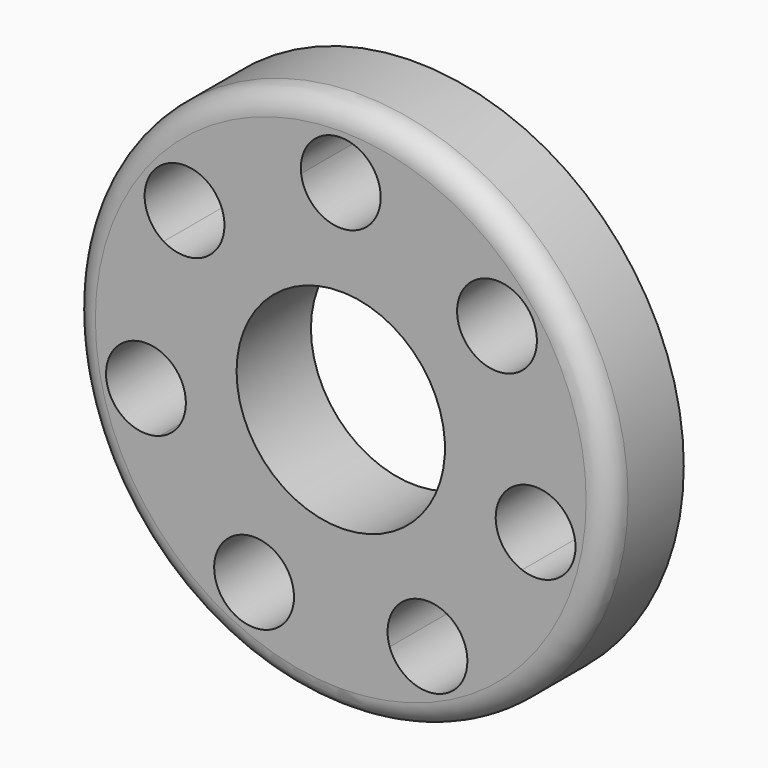
from build123d import *

# Parameters (mm, degrees)
F0_R     = 73.4225499851
F1_DEPTH = 25.4
F3_R     = 6.35
F5_DEPTH = 25.4
F6_R     = 28.4745991817
F7_DEPTH = 25.4


with BuildPart() as f1:
    # F0 (on Front) → F1 (new body)
    with BuildSketch(Plane.XZ):
        Circle(F0_R)
    extrude(amount=F1_DEPTH)

    # F3
    f3_edges = [f1.edges().sort_by_distance(p)[0] for p in [
        (-73.42255, -25.4, 0),
    ]]
    fillet(f3_edges, radius=F3_R)

    # F4 (on face) → F5 (cut)
    with BuildSketch(Plane.XZ.offset(25.4)):
        with BuildLine():
            ThreePointArc((10.828438703, 53.2833849069), (10.8892176697, 53.9458802451), (10.9095024699, 54.6108484268))
            ThreePointArc((10.9095024699, 54.6108484268), (-0.6649681817, 65.5000660965), (-10.828438703, 53.2833849069))
            ThreePointArc((-10.828438703, 53.2833849069), (0, 54.3725499851), (10.828438703, 53.2833849069))
        make_face()
        with BuildLine():
            ThreePointArc((10.828438703, 53.2833849069), (0, 54.3725499851), (-10.828438703, 53.2833849069))
            ThreePointArc((-10.828438703, 53.2833849069), (0, 43.7013459569), (10.828438703, 53.2833849069))
        make_face()
        with BuildLine():
            ThreePointArc((-48.4100489141, 24.7556328141), (-42.5101713604, 33.9007304168), (-34.9072067114, 41.6876613819))
            ThreePointArc((-34.9072067114, 41.6876613819), (-51.2258730734, 40.8512705983), (-48.4100489141, 24.7556328141))
        make_face()
        with BuildLine():
            ThreePointArc((-31.7869781145, 34.049307065), (-32.5971155871, 38.1748459137), (-34.9072067114, 41.6876613819))
            ThreePointArc((-34.9072067114, 41.6876613819), (-42.5101713604, 33.9007304168), (-48.4100489141, 24.7556328141))
            ThreePointArc((-48.4100489141, 24.7556328141), (-37.3727104759, 24.5269798299), (-31.7869781145, 34.049307065))
        make_face()
        with BuildLine():
            ThreePointArc((48.4100489141, 24.7556328141), (42.5101713604, 33.9007304168), (34.9072067114, 41.6876613819))
            ThreePointArc((34.9072067114, 41.6876613819), (34.1670880954, 27.2473435317), (48.4100489141, 24.7556328141))
        make_face()
        with BuildLine():
            ThreePointArc((53.6059830542, 34.049307065), (46.8220194331, 44.1486720622), (34.9072067114, 41.6876613819))
            ThreePointArc((34.9072067114, 41.6876613819), (42.5101713604, 33.9007304168), (48.4100489141, 24.7556328141))
            ThreePointArc((48.4100489141, 24.7556328141), (52.2188078195, 28.7255369565), (53.6059830542, 34.049307065))
        make_face()
        with BuildLine():
            ThreePointArc((-49.5379049078, -22.4136157107), (-53.009316637, -12.0990306043), (-54.3570134948, -1.299721437))
            ThreePointArc((-54.3570134948, -1.299721437), (-63.8776189051, -14.5796496747), (-49.5379049078, -22.4136157107))
        make_face()
        with BuildLine():
            ThreePointArc((-42.3321379694, -12.1520569961), (-45.9324312127, -4.0531246824), (-54.3570134948, -1.299721437))
            ThreePointArc((-54.3570134948, -1.299721437), (-53.009316637, -12.0990306043), (-49.5379049078, -22.4136157107))
            ThreePointArc((-49.5379049078, -22.4136157107), (-44.3135063658, -18.421480104), (-42.3321379694, -12.1520569961))
        make_face()
        with BuildLine():
            ThreePointArc((49.5379049078, -22.4136157107), (53.009316637, -12.0990306043), (54.3570134948, -1.299721437))
            ThreePointArc((54.3570134948, -1.299721437), (42.6056619733, -9.7244643175), (49.5379049078, -22.4136157107))
        make_face()
        with BuildLine():
            ThreePointArc((64.1511429091, -12.1520569961), (61.340572753, -4.8428477695), (54.3570134948, -1.299721437))
            ThreePointArc((54.3570134948, -1.299721437), (53.009316637, -12.0990306043), (49.5379049078, -22.4136157107))
            ThreePointArc((49.5379049078, -22.4136157107), (59.5110635472, -21.0801910696), (64.1511429091, -12.1520569961))
        make_face()
        with BuildLine():
            ThreePointArc((-13.3627081169, -52.7049544509), (-23.5913652929, -48.9879748051), (-32.8748804356, -43.3083875044))
            ThreePointArc((-32.8748804356, -43.3083875044), (-28.4282148354, -59.031796372), (-13.3627081169, -52.7049544509))
        make_face()
        with BuildLine():
            ThreePointArc((-12.7852566419, -49.2026742823), (-20.6233841848, -38.7344413752), (-32.8748804356, -43.3083875044))
            ThreePointArc((-32.8748804356, -43.3083875044), (-23.5913652929, -48.9879748051), (-13.3627081169, -52.7049544509))
            ThreePointArc((-13.3627081169, -52.7049544509), (-12.930587523, -50.9774571271), (-12.7852566419, -49.2026742823))
        make_face()
        with BuildLine():
            ThreePointArc((13.3627081169, -52.7049544509), (23.5913652929, -48.9879748051), (32.8748804356, -43.3083875044))
            ThreePointArc((32.8748804356, -43.3083875044), (18.9613033883, -39.3735521926), (13.3627081169, -52.7049544509))
        make_face()
        with BuildLine():
            ThreePointArc((34.6042615817, -49.2026742823), (34.1629920189, -46.1312993553), (32.8748804356, -43.3083875044))
            ThreePointArc((32.8748804356, -43.3083875044), (23.5913652929, -48.9879748051), (13.3627081169, -52.7049544509))
            ThreePointArc((13.3627081169, -52.7049544509), (25.4695419566, -59.9668458711), (34.6042615817, -49.2026742823))
        make_face()
    extrude(amount=-F5_DEPTH, mode=Mode.SUBTRACT)

    # F6 (on face) → F7 (cut)
    with BuildSketch(Plane(origin=(0, 0, 0), x_dir=(-1, 0, 0), z_dir=(0, 1, 0))):
        Circle(F6_R)
    extrude(amount=-F7_DEPTH, mode=Mode.SUBTRACT)


solid = f1.part
